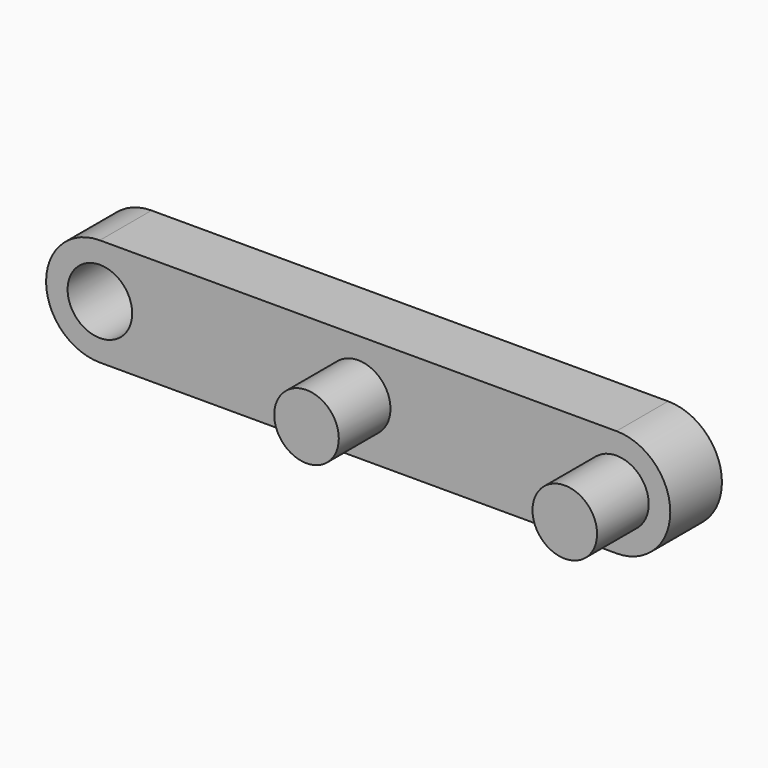
from build123d import *

# Parameters (mm, degrees)
F0_R     = 9.525
F1_DEPTH = 9.525
F2_R     = 9.525
F3_DEPTH = 19.05


# Not quite as in the source:
# - a feature of the source that left no trace in its solid (it failed there, or was rolled back) is left out
# - a pattern or mirror of a feature is missing from the dataset's text; its kind, count and spacing are read off the source's solid


with BuildPart() as f1:
    # F0 (on Front) → F1 (new body, symmetric)
    with BuildSketch(Plane.XZ):
        with BuildLine():
            ThreePointArc((76.2, -15.875), (92.075, 0), (76.2, 15.875))
            Line((76.2, 15.875), (-76.2, 15.875))
            ThreePointArc((-76.2, 15.875), (-92.075, 0), (-76.2, -15.875))
            Line((-76.2, -15.875), (76.2, -15.875))
        make_face()
        with Locations((-76.2, 0)):
            Circle(F0_R, mode=Mode.SUBTRACT)
        with Locations((76.2, 0)):
            Circle(F0_R, mode=Mode.SUBTRACT)
        with Locations((76.2, 0)):
            Circle(F0_R)
    extrude(amount=F1_DEPTH, both=True)

    # F2 (on face) → F3 (join)
    with BuildSketch(Plane.XZ.offset(9.525)):
        Circle(F2_R)
    f3 = extrude(amount=F3_DEPTH)

    # F3_copies: F3 across plane
    add(f3.mirror(Plane(origin=(38.1, 0, 0), x_dir=(0, 0, 1), z_dir=(1, 0, 0))))


solid = f1.part
